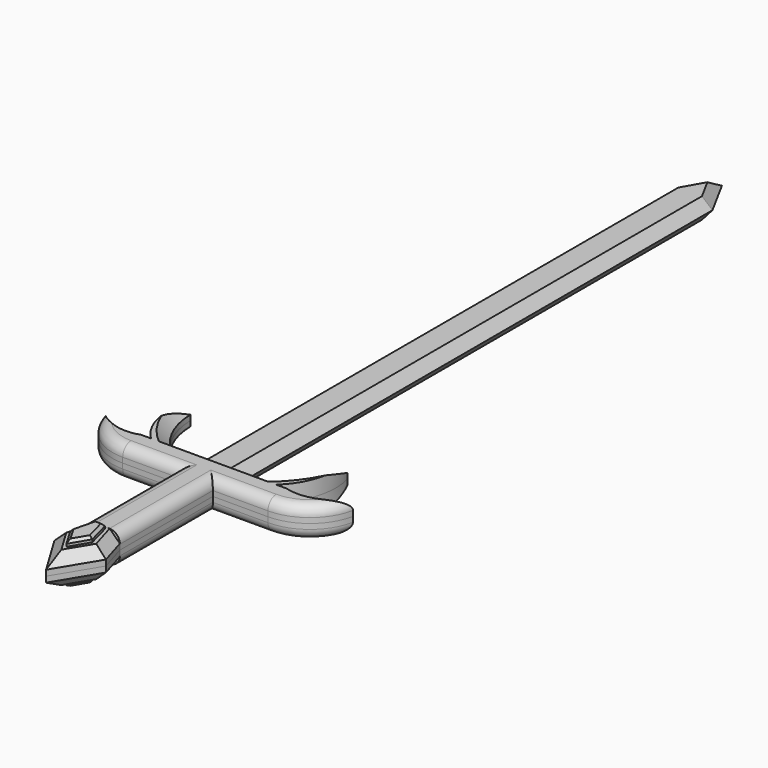
from build123d import *

# Parameters (mm, degrees)
F0_W        = 16.9903710485
F0_H        = 11.2329293042
F0_H_2      = 56.7607395351
F1_DEPTH    = 7.62
F2_R        = 5.08
F4_DEPTH    = 5.08
F5_T1_DEPTH = 332.8395862184
F5_T3_DEPTH = 332.7291762168
F5_T5_DEPTH = 64.4306283308
F5_T7_DEPTH = 64.1781797191
F6_R        = 5.08
F7_SIZE     = 5.08
F9_DEPTH    = 7.62
F10_SIZE    = 4.826
F12_DEPTH   = 2.54
F13_SIZE    = 1.27


# Not quite as in the source:
# - a fillet or chamfer that OpenCascade refuses, or shapes differently, is made with other operations: its cross-section is extruded or revolved along the edge and cut away or added


with BuildPart() as f1:
    # F0 (on Top) → F1 (new body)
    with BuildSketch(Plane.XY):
        with Locations((-4.2698672041, -32.2207761928)):
            Rectangle(F0_W, F0_H)
        Polygon((-12.7650527284, -37.837240845), (-12.7650527284, -26.6043115407), (-22.2795344889, -26.6043115407), (-34.9734351039, -26.6043115407), (-39.8079305887, -26.6043115407), (-39.8079305887, -37.837240845), align=None)
        Polygon((13.4834656492, -26.6043115407), (4.2253183201, -26.6043115407), (4.2253183201, -37.837240845), (31.1368945986, -37.837240845), (31.1368945986, -26.6043115407), (26.1162724346, -26.6043115407), align=None)
        with Locations((-4.2698672041, -66.2176106125)):
            Rectangle(F0_W, F0_H_2)
        with BuildLine():
            Line((-34.9734351039, -26.6043115407), (-22.2795344889, -26.6043115407))
            ThreePointArc((-22.2795344889, -26.6043115407), (-36.2117622733, -13.0200039257), (-41.5752306581, 5.6849042885))
            ThreePointArc((-41.5752306581, 5.6849042885), (-43.2880257194, -11.4847943334), (-34.9734351039, -26.6043115407))
        make_face()
        with BuildLine():
            ThreePointArc((35.2943129838, 5.6849042885), (27.9247695922, -12.8481340326), (13.4834656492, -26.6043115407))
            Line((13.4834656492, -26.6043115407), (26.1162724346, -26.6043115407))
            ThreePointArc((26.1162724346, -26.6043115407), (35.3252385886, -11.7728990546), (35.2943129838, 5.6849042885))
        make_face()
        with BuildLine():
            ThreePointArc((-64.1463175416, -17.3298995942), (-55.7210393724, -32.026898994), (-39.8079305887, -37.837240845))
            Line((-39.8079305887, -37.837240845), (-39.8079305887, -26.6043115407))
            ThreePointArc((-39.8079305887, -26.6043115407), (-53.6778361214, -26.4302012719), (-64.1463175416, -17.3298995942))
        make_face()
        with BuildLine():
            Line((31.1368945986, -26.6043115407), (31.1368945986, -37.837240845))
            ThreePointArc((31.1368945986, -37.837240845), (47.3595070101, -32.0602618252), (56.2793202698, -17.3298995942))
            ThreePointArc((56.2793202698, -17.3298995942), (45.2099392934, -26.038489943), (31.1368945986, -26.6043115407))
        make_face()
    extrude(amount=F1_DEPTH)

    # F2
    f2_edges = [f1.edges().sort_by_distance(p)[0] for p in [
        (-12.765053, -66.217611, 7.62),
        (4.225318, -66.217611, 7.62),
    ]]
    fillet(f2_edges, radius=F2_R)

    # F6
    f6_edges = [f1.edges().sort_by_distance(p)[0] for p in [
        (-26.286492, -37.837241, 7.62),
        (17.681106, -37.837241, 7.62),
        (-55.721039, -32.026899, 7.62),
        (47.359507, -32.060262, 7.62),
    ]]
    fillet(f6_edges, radius=F6_R)

    # F7
    f7_edges = [f1.edges().sort_by_distance(p)[0] for p in [
        (-36.211762, -13.020004, 7.62),
        (27.92477, -12.848134, 7.62),
    ]]
    chamfer(f7_edges, length=F7_SIZE)


with BuildPart() as f4:
    # F3 (on Top) → F4 (new body)
    with BuildSketch(Plane.XY):
        Polygon((-16.8165620416, 266.4132416248), (-16.8165620416, -27.1466755785), (7.4740615673, -27.036265577), (7.4740615673, 266.4132416248), (-4.4111721218, 288.2919311523), align=None)
    extrude(amount=F4_DEPTH)

    # F5: chamfer of 7.62 x 6.3939391896 on 4 edges, made by hand

    # F5_s2 → F5_t1 (cut)
    with BuildSketch(Plane.XZ.offset(-286.0530761323)):
        Polygon((-16.8165620416, -2.54), (-10.4226228521, 5.08), (-16.8165620416, 5.08), align=None)
    extrude(amount=F5_T1_DEPTH, mode=Mode.SUBTRACT)

    # F5_s4 → F5_t3 (cut)
    with BuildSketch(Plane.XZ.offset(-286.0530761323)):
        Polygon((7.4740615673, -2.54), (1.0801223778, 5.08), (7.4740615673, 5.08), align=None)
    extrude(amount=F5_T3_DEPTH, mode=Mode.SUBTRACT)

    # F5_s6 → F5_t5 (cut)
    with BuildSketch(Plane(origin=(132.309777211, 233.3473236835, 0), x_dir=(0, 0, 1), z_dir=(-0.4932372465, -0.869894832, 0))):
        Polygon((-2.54, 146.0335741426), (5.08, 139.6396349531), (5.08, 146.0335741426), align=None)
    extrude(amount=F5_T5_DEPTH, mode=Mode.SUBTRACT)

    # F5_s8 → F5_t7 (cut)
    with BuildSketch(Plane(origin=(-100.6695105648, 185.3154110511, 0), x_dir=(0, 0, 1), z_dir=(-0.4773471727, 0.8787147869, 0))):
        Polygon((-2.54, 133.7391760771), (5.08, 127.3452368875), (5.08, 133.7391760771), align=None)
    extrude(amount=F5_T7_DEPTH, mode=Mode.SUBTRACT)


with BuildPart() as f9:
    # F8 (on Top) → F9 (new body)
    with BuildSketch(Plane.XY):
        Polygon((4.2217592709, -94.6217030287), (-12.7686117776, -94.6217030287), (-16.8529637158, -108.2521602511), (-4.2734262533, -129.0639638901), (8.2952212542, -108.2521602511), align=None)
    extrude(amount=F9_DEPTH)

    # F10
    f10_edges = [f9.edges().sort_by_distance(p)[0] for p in [
        (-10.563195, -118.658062, 7.62),
        (2.010898, -118.658062, 7.62),
        (-14.810788, -101.436932, 7.62),
        (6.25849, -101.436932, 7.62),
    ]]
    chamfer(f10_edges, length=F10_SIZE)


with BuildPart() as f12:
    # F11 (on face) → F12 (new body)
    with BuildSketch(Plane.XY.offset(7.62)):
        Polygon((-4.2752149429, -116.7355105281), (1.1395043943, -107.5873051191), (-1.9756610023, -96.0157086394), (-6.6725995569, -96.0157086394), (-9.5803312475, -107.5873051191), align=None)
    extrude(amount=F12_DEPTH)

    # F13
    f13_edges = [f12.edges().sort_by_distance(p)[0] for p in [
        (-8.126465, -101.801507, 10.16),
        (-4.32413, -96.015709, 10.16),
        (-0.418078, -101.801507, 10.16),
        (-1.567855, -112.161408, 10.16),
        (-6.927773, -112.161408, 10.16),
    ]]
    chamfer(f13_edges, length=F13_SIZE)


with BuildPart() as f14_1:
    # F14: instance of F4
    add(f4.part.mirror(Plane.XY))


with BuildPart() as f14_2:
    # F14: instance of F1
    add(f1.part.mirror(Plane.XY))


with BuildPart() as f14_3:
    # F14: instance of F12
    add(f12.part.mirror(Plane.XY))


with BuildPart() as f14_4:
    # F14: instance of F9
    add(f9.part.mirror(Plane.XY))


solid = Compound([f1.part, f4.part, f9.part, f12.part, f14_1.part, f14_2.part, f14_3.part, f14_4.part])
